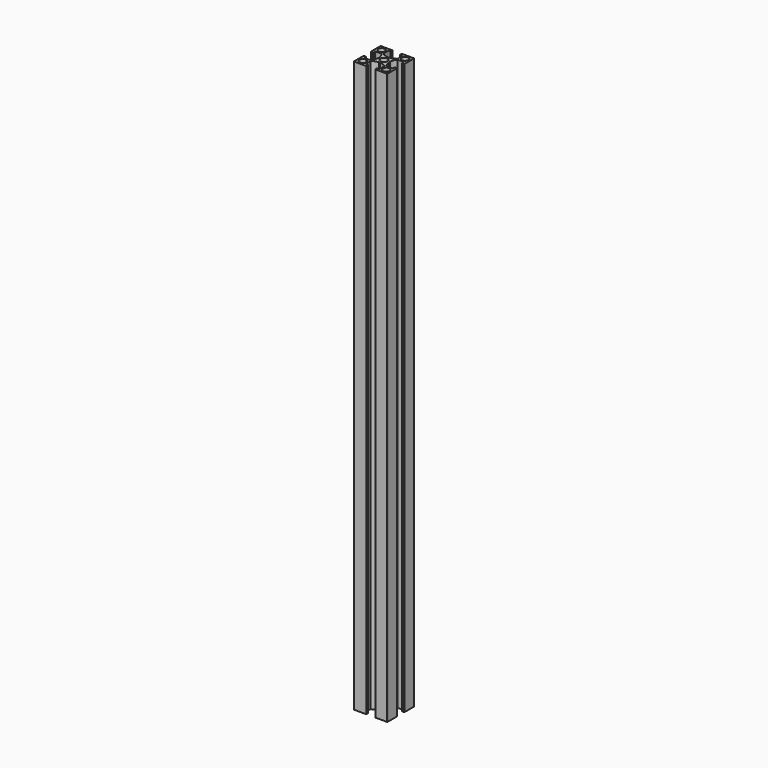
from build123d import *

# Parameters (mm, degrees)
F1_DEPTH = 340


# Not quite as in the source:
# - ends of sketch curves that miss each other by under 0.0002 mm in the source are joined


with BuildPart() as f1:
    # F0 (on Top) → F1 (new body)
    with BuildSketch(Plane.XY):
        with BuildLine():
            ThreePointArc((-2.15, 0), (-1.5202795796, 1.5202795796), (0, 2.15))
            Line((0, 2.15), (0, 3))
            Line((0, 3), (-0.307277, 3.307278))
            ThreePointArc((-0.307277, 3.307278), (-2.2820211583, 3.7143800615), (-4.036565823, 4.7078182229))
            ThreePointArc((-4.036565823, 4.7078182229), (-4.1201572004, 4.8123081084), (-4.15, 4.94275))
            Line((-4.15, 4.94275), (-4.15, 8.2))
            ThreePointArc((-4.15, 8.2), (-4.0621320344, 8.4121320344), (-3.85, 8.5))
            Line((-3.85, 8.5), (-2.95, 8.5))
            ThreePointArc((-2.95, 8.5), (-2.7378679656, 8.5878679656), (-2.65, 8.8))
            Line((-2.65, 8.8), (-2.65, 9.7))
            ThreePointArc((-2.65, 9.7), (-2.7378679656, 9.9121320344), (-2.95, 10))
            Line((-2.95, 10), (-9.7, 10))
            ThreePointArc((-9.7, 10), (-9.9121320344, 9.9121320344), (-10, 9.7))
            Line((-10, 9.7), (-10, 2.95))
            ThreePointArc((-10, 2.95), (-9.9121320344, 2.7378679656), (-9.7, 2.65))
            Line((-9.7, 2.65), (-8.8, 2.65))
            ThreePointArc((-8.8, 2.65), (-8.5878679656, 2.7378679656), (-8.5, 2.95))
            Line((-8.5, 2.95), (-8.5, 3.85))
            ThreePointArc((-8.5, 3.85), (-8.4121320344, 4.0621320344), (-8.2, 4.15))
            Line((-8.2, 4.15), (-4.942749, 4.15))
            ThreePointArc((-4.942749, 4.15), (-4.812307461, 4.1201573706), (-4.7078173786, 4.0365666993))
            ThreePointArc((-4.7078173786, 4.0365666993), (-3.7143793747, 2.2820219924), (-3.3072773955, 0.3072779813))
            Line((-3.3072773955, 0.3072779813), (-3, 0))
            Line((-3, 0), (-2.15, 0))
        make_face()
        with BuildLine():
            ThreePointArc((-7, 5), (-8.4142135624, 5.5857864376), (-9, 7))
            ThreePointArc((-9, 7), (-8.4142135624, 8.4142135624), (-7, 9))
            ThreePointArc((-7, 9), (-5.5857864376, 8.4142135624), (-5, 7))
            ThreePointArc((-5, 7), (-5.5857864376, 5.5857864376), (-7, 5))
        make_face(mode=Mode.SUBTRACT)
        with BuildLine():
            ThreePointArc((0, 2.15), (1.5202795796, 1.5202795796), (2.15, 0))
            Line((2.15, 0), (3, 0))
            Line((3, 0), (3.307278, 0.307278))
            ThreePointArc((3.307278, 0.307278), (3.7143803747, 2.2820219924), (4.7078187099, 4.0365664363))
            ThreePointArc((4.7078187099, 4.0365664363), (4.812308461, 4.1201573706), (4.94275, 4.15))
            Line((4.94275, 4.15), (8.2, 4.15))
            ThreePointArc((8.2, 4.15), (8.4121320344, 4.0621320344), (8.5, 3.85))
            Line((8.5, 3.85), (8.5, 2.95))
            ThreePointArc((8.5, 2.95), (8.5878679656, 2.7378679656), (8.8, 2.65))
            Line((8.8, 2.65), (9.7, 2.65))
            ThreePointArc((9.7, 2.65), (9.9121320344, 2.7378679656), (10, 2.95))
            Line((10, 2.95), (10, 9.7))
            ThreePointArc((10, 9.7), (9.9121320344, 9.9121320344), (9.7, 10))
            Line((9.7, 10), (2.95, 10))
            ThreePointArc((2.95, 10), (2.7378679656, 9.9121320344), (2.65, 9.7))
            Line((2.65, 9.7), (2.65, 8.8))
            ThreePointArc((2.65, 8.8), (2.7378679656, 8.5878679656), (2.95, 8.5))
            Line((2.95, 8.5), (3.85, 8.5))
            ThreePointArc((3.85, 8.5), (4.0621320344, 8.4121320344), (4.15, 8.2))
            Line((4.15, 8.2), (4.15, 4.94275))
            ThreePointArc((4.15, 4.94275), (4.1201572004, 4.8123081084), (4.036566086, 4.7078178916))
            ThreePointArc((4.036566086, 4.7078178916), (2.2820216259, 3.7143802371), (0.3072779813, 3.3072783955))
            Line((0.3072779813, 3.3072783955), (0, 3))
            Line((0, 3), (0, 2.15))
        make_face()
        with BuildLine():
            ThreePointArc((7, 9), (8.4142135624, 8.4142135624), (9, 7))
            ThreePointArc((9, 7), (8.4142135624, 5.5857864376), (7, 5))
            ThreePointArc((7, 5), (5.5857864376, 5.5857864376), (5, 7))
            ThreePointArc((5, 7), (5.5857864376, 8.4142135624), (7, 9))
        make_face(mode=Mode.SUBTRACT)
        with BuildLine():
            Line((3, 0), (2.15, 0))
            ThreePointArc((2.15, 0), (1.5202795796, -1.5202795796), (0, -2.15))
            Line((0, -2.15), (0, -3))
            Line((0, -3), (0.307278, -3.307277))
            ThreePointArc((0.307278, -3.307277), (2.2820216259, -3.7143792371), (4.036565823, -4.7078172229))
            ThreePointArc((4.036565823, -4.7078172229), (4.1201572004, -4.8123071084), (4.15, -4.942749))
            Line((4.15, -4.942749), (4.15, -8.2))
            ThreePointArc((4.15, -8.2), (4.0621320344, -8.4121320344), (3.85, -8.5))
            Line((3.85, -8.5), (2.95, -8.5))
            ThreePointArc((2.95, -8.5), (2.7378679656, -8.5878679656), (2.65, -8.8))
            Line((2.65, -8.8), (2.65, -9.7))
            ThreePointArc((2.65, -9.7), (2.7378679656, -9.9121320344), (2.95, -10))
            Line((2.95, -10), (9.7, -10))
            ThreePointArc((9.7, -10), (9.9121320344, -9.9121320344), (10, -9.7))
            Line((10, -9.7), (10, -2.95))
            ThreePointArc((10, -2.95), (9.9121320344, -2.7378679656), (9.7, -2.65))
            Line((9.7, -2.65), (8.8, -2.65))
            ThreePointArc((8.8, -2.65), (8.5878679656, -2.7378679656), (8.5, -2.95))
            Line((8.5, -2.95), (8.5, -3.85))
            ThreePointArc((8.5, -3.85), (8.4121320344, -4.0621320344), (8.2, -4.15))
            Line((8.2, -4.15), (4.94275, -4.15))
            ThreePointArc((4.94275, -4.15), (4.8123081084, -4.1201572004), (4.7078178916, -4.036566086))
            ThreePointArc((4.7078178916, -4.036566086), (3.7143800615, -2.2820211583), (3.3072783483, -0.3072769835))
            Line((3.3072783483, -0.3072769835), (3, 0))
        make_face()
        with BuildLine():
            ThreePointArc((7, -5), (8.4142135624, -5.5857864376), (9, -7))
            ThreePointArc((9, -7), (8.4142135624, -8.4142135624), (7, -9))
            ThreePointArc((7, -9), (5.5857864376, -8.4142135624), (5, -7))
            ThreePointArc((5, -7), (5.5857864376, -5.5857864376), (7, -5))
        make_face(mode=Mode.SUBTRACT)
        with BuildLine():
            Line((0, -3), (0, -2.15))
            ThreePointArc((0, -2.15), (-1.5202795796, -1.5202795796), (-2.15, 0))
            Line((-2.15, 0), (-3, 0))
            Line((-3, 0), (-3.307277, -0.307277))
            ThreePointArc((-3.307277, -0.307277), (-3.7143790615, -2.2820211583), (-4.7078172229, -4.036565823))
            ThreePointArc((-4.7078172229, -4.036565823), (-4.8123071084, -4.1201572004), (-4.942749, -4.15))
            Line((-4.942749, -4.15), (-8.2, -4.15))
            ThreePointArc((-8.2, -4.15), (-8.4121320344, -4.0621320344), (-8.5, -3.85))
            Line((-8.5, -3.85), (-8.5, -2.95))
            ThreePointArc((-8.5, -2.95), (-8.5878679656, -2.7378679656), (-8.8, -2.65))
            Line((-8.8, -2.65), (-9.7, -2.65))
            ThreePointArc((-9.7, -2.65), (-9.9121320344, -2.7378679656), (-10, -2.95))
            Line((-10, -2.95), (-10, -9.7))
            ThreePointArc((-10, -9.7), (-9.9121320344, -9.9121320344), (-9.7, -10))
            Line((-9.7, -10), (-2.95, -10))
            ThreePointArc((-2.95, -10), (-2.7378679656, -9.9121320344), (-2.65, -9.7))
            Line((-2.65, -9.7), (-2.65, -8.8))
            ThreePointArc((-2.65, -8.8), (-2.7378679656, -8.5878679656), (-2.95, -8.5))
            Line((-2.95, -8.5), (-3.85, -8.5))
            ThreePointArc((-3.85, -8.5), (-4.0621320344, -8.4121320344), (-4.15, -8.2))
            Line((-4.15, -8.2), (-4.15, -4.942749))
            ThreePointArc((-4.15, -4.942749), (-4.1201572004, -4.8123071084), (-4.036566086, -4.7078168916))
            ThreePointArc((-4.036566086, -4.7078168916), (-2.2820211583, -3.7143790615), (-0.3072769835, -3.3072773483))
            Line((-0.3072769835, -3.3072773483), (0, -3))
        make_face()
        with BuildLine():
            ThreePointArc((-7, -9), (-8.4142135624, -8.4142135624), (-9, -7))
            ThreePointArc((-9, -7), (-8.4142135624, -5.5857864376), (-7, -5))
            ThreePointArc((-7, -5), (-5.5857864376, -5.5857864376), (-5, -7))
            ThreePointArc((-5, -7), (-5.5857864376, -8.4142135624), (-7, -9))
        make_face(mode=Mode.SUBTRACT)
    extrude(amount=F1_DEPTH)


solid = f1.part
